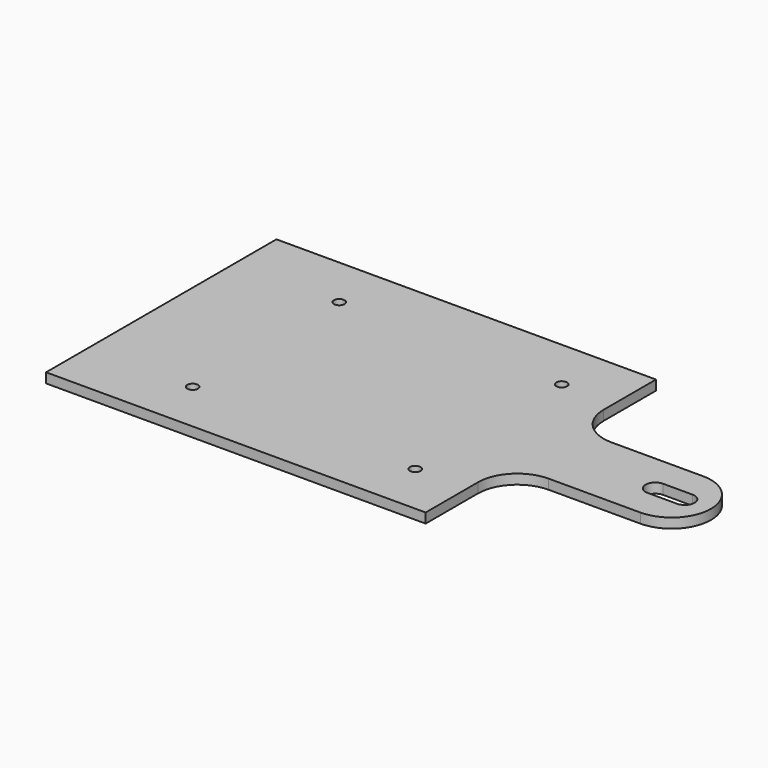
from build123d import *

# Parameters (mm, degrees)
F1_DEPTH = 9.525
F2_DEPTH = 9.525
F4_D     = 10.31875


# Not quite as in the source:
# - a feature of the source that left no trace in its solid (it failed there, or was rolled back) is left out


with BuildPart() as f1:
    # F0 (on Top) → F1 (new body)
    with BuildSketch(Plane.XY):
        Polygon((-266.7, -139.7), (101.6, -139.7), (101.6, -76.2), (101.6, 76.2), (101.6, 139.7), (-266.7, 139.7), align=None)
    extrude(amount=F1_DEPTH)

    # F0 (on Top) → F2 (join)
    with BuildSketch(Plane.XY):
        with BuildLine():
            Line((101.6, 76.2), (101.6, -76.2))
            ThreePointArc((101.6, -76.2), (112.7592316368, -49.2592316368), (139.7, -38.1))
            Line((139.7, -38.1), (228.6, -38.1))
            ThreePointArc((228.6, -38.1), (266.7, 0), (228.6, 38.1))
            Line((228.6, 38.1), (139.7, 38.1))
            ThreePointArc((139.7, 38.1), (112.7592316368, 49.2592316368), (101.6, 76.2))
        make_face()
        with BuildLine():
            Line((212.725, 9.525), (241.3, 9.525))
            ThreePointArc((241.3, 9.525), (250.825, 0), (241.3, -9.525))
            Line((241.3, -9.525), (212.725, -9.525))
            ThreePointArc((212.725, -9.525), (203.2, 0), (212.725, 9.525))
        make_face(mode=Mode.SUBTRACT)
    extrude(amount=F2_DEPTH)

    # F4 (through all)
    with Locations(Plane(origin=(0, 0, 0), x_dir=(1, 0, 0), z_dir=(0, 0, -1))):
        with Locations((-165.1, -88.9), (-165.1, 88.9), (50.8, 88.9), (50.8, -88.9)):
            Hole(F4_D / 2)


solid = f1.part
